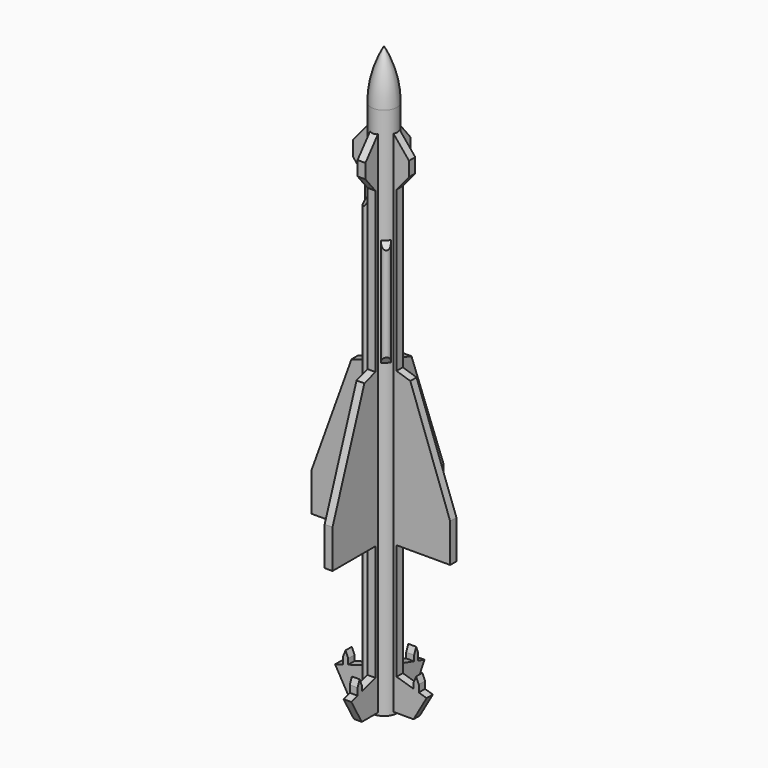
from build123d import *

# Parameters (mm, degrees)
F4_DEPTH  = 0.1
F5_COUNT  = 4
F8_DEPTH  = 10.8333333333
F11_DEPTH = 2.4
F12_SIZE2 = 0.09999
F12_SIZE  = 0.173195


# Not quite as in the source:
# - a fillet or chamfer is up to 0.001 mm smaller than in the source, because OpenCascade refuses the exact size


with BuildPart() as f2:
    # F1 (on Front) → F2 (revolve)
    with BuildSketch(Plane.XZ):
        with BuildLine():
            Line((0, 14.8666666667), (0, 0))
            Line((0, 0), (0.3333333333, 0))
            Line((0.3333333333, 0), (0.3333333333, 13.6))
            ThreePointArc((0.3333333333, 13.6), (0.2486051426, 14.2548960901), (0, 14.8666666667))
        make_face()
    revolve(axis=Axis((0, 0, 7.4333333333), (0, 0, 1)))

    # F3 (on Front) → F4 (join, symmetric)
    with BuildSketch(Plane.XZ):
        Polygon((0, 13.4391304348), (0, 0.0666666667), (0.8333333333, 0.0666666667), (1.1666666667, 0.65), (0.9666666667, 0.71), (0.8333333333, 0.75), (0.4, 0.88), (0.4, 3.8333333333), (1.7666666667, 3.8333333333), (1.7666666667, 4.8166666667), (0.75, 7.6333333333), (0.4, 7.7453333333), (0.4, 11.8144927536), (0.7166666667, 12.2), (0.7166666667, 12.5666666667), align=None)
        Polygon((0.8333333333, 0.75), (0.9666666667, 0.71), (0.9666666667, 0.8890524292), (0.9, 1.05), (0.8333333333, 0.8890524292), align=None)
    extrude(amount=F4_DEPTH, both=True)

    # F5: F2 ×4 about axis
    f5_axis = Axis((0, 0, 0), (0, 0, 1))


with BuildPart() as f2_1:
    add(f2.part)
    for i in range(1, F5_COUNT):
        add(f2.part.rotate(f5_axis, i * 360 / F5_COUNT))

    # F7 (on offset) → F8 (join)
    with BuildSketch(Plane.XY.offset(0.4666666667)):
        with BuildLine():
            Line((-0.1110620592, 0.030359297), (-0.3064129385, -0.1649915823))
            ThreePointArc((-0.3064129385, -0.1649915823), (-0.3064129385, -0.3064129385), (-0.1649915823, -0.3064129385))
            Line((-0.1649915823, -0.3064129385), (0.030359297, -0.1110620592))
            Line((0.030359297, -0.1110620592), (-0.1110620592, 0.030359297))
        make_face()
    extrude(amount=F8_DEPTH)

    # F10 (on offset) → F11 (join)
    with BuildSketch(Plane.XY.offset(8.1)):
        with BuildLine():
            Line((0.1737662231, -0.0323448669), (0.0323448669, -0.1737662231))
            Line((0.0323448669, -0.1737662231), (0.1649915823, -0.3064129385))
            ThreePointArc((0.1649915823, -0.3064129385), (0.3064129385, -0.3064129385), (0.3064129385, -0.1649915823))
            Line((0.3064129385, -0.1649915823), (0.1737662231, -0.0323448669))
        make_face()
    extrude(amount=F11_DEPTH)

    # F12 (call 1 of 4: OpenCascade refuses the feature's edges together) (size 0.1732050808 and 0.1 in the source; OpenCascade refuses exactly that, so slightly less here)
    f12_edges = [f2_1.edges().sort_by_distance(p)[0] for p in [
        (-0.235702, -0.235702, 11.3),
    ]]
    f12_side = f2_1.faces().sort_by_distance((-0.333333, 0, 0.013633))[0]
    chamfer(f12_edges, length=F12_SIZE, length2=F12_SIZE2, reference=f12_side)

    # F12#2 (call 2 of 4) (size 0.1732050808 and 0.1 in the source; OpenCascade refuses exactly that, so slightly less here)
    f12_2_edges = [f2_1.edges().sort_by_distance(p)[0] for p in [
        (-0.235702, -0.235702, 0.466667),
    ]]
    f12_2_side = f2_1.faces().sort_by_distance((-0.333333, 0, 0.013633))[0]
    chamfer(f12_2_edges, length=F12_SIZE, length2=F12_SIZE2, reference=f12_2_side)

    # F12#3 (call 3 of 4) (size 0.1732050808 and 0.1 in the source; OpenCascade refuses exactly that, so slightly less here)
    f12_3_edges = [f2_1.edges().sort_by_distance(p)[0] for p in [
        (0.235702, -0.235702, 8.1),
    ]]
    f12_3_side = f2_1.faces().sort_by_distance((-0.333333, 0, 0.013633))[0]
    chamfer(f12_3_edges, length=F12_SIZE, length2=F12_SIZE2, reference=f12_3_side)

    # F12#4 (call 4 of 4) (size 0.1732050808 and 0.1 in the source; OpenCascade refuses exactly that, so slightly less here)
    f12_4_edges = [f2_1.edges().sort_by_distance(p)[0] for p in [
        (0.235702, -0.235702, 10.5),
    ]]
    f12_4_side = f2_1.faces().sort_by_distance((-0.333333, 0, 0.013633))[0]
    chamfer(f12_4_edges, length=F12_SIZE, length2=F12_SIZE2, reference=f12_4_side)


solid = f2_1.part
